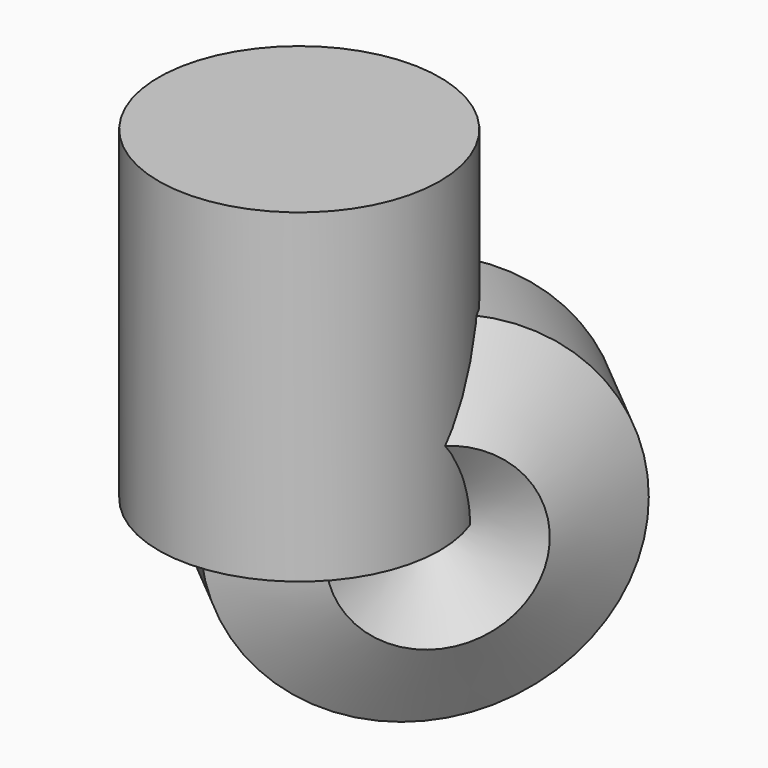
from build123d import *

# Parameters (mm, degrees)
F0_R     = 54.9531653684
F1_DEPTH = 127
F7_DEPTH = 25.4


# Not quite as in the source:
# - a feature of the source that left no trace in its solid (it failed there, or was rolled back) is left out
# - the program builds the solid bodies; features that only make, move or delete a surface that nothing else refers to are left out


with BuildPart() as f1:
    # F0 (on Top) → F1 (new body)
    with BuildSketch(Plane.XY):
        Circle(F0_R)
    extrude(amount=F1_DEPTH)


with BuildPart() as f3:
    # F2 (on Top) → F3 (revolve)
    with BuildSketch(Plane.XY):
        Polygon((30.9442904428, -25.8326890354), (37.8439101741, 13.8821971078), (6.8996197313, 39.7148861432), (-30.9442904428, 25.8326890354), (-37.8439101741, -13.8821971078), (-6.8996197313, -39.7148861432), align=None)
    revolve(axis=Axis((22.3717649527, 26.7985416255, 0), (0.7676624397, -0.640854413, 0)))


with BuildPart() as f7:
    # F6 (on Top) → F7 (new body)
    with BuildSketch(Plane.XY):
        with BuildLine():
            add(Edge.make_bspline(
                [(-22.4183332175, 16.1747615784), (-11.8871169461, 25.9707679053), (-5.6486125726, 51.1465707181), (42.7874188306, 27.4433614183), (39.8462276715, -30.123574606), (-2.9479560075, -20.4408335204), (-31.1948387365, -43.0855866328), (-18.3031677908, -3.1092882088), (-65.8787672835, -7.2071620203), (-32.9625958172, 6.3666197193), (-22.4183332175, 16.1747615784)],
                knots=[0, 0, 0, 0, 0.1298859642, 0.2693514147, 0.414375979, 0.5513899534, 0.6555656862, 0.7633147629, 0.8699531299, 1, 1, 1, 1], degree=3))
        make_face()
    extrude(amount=F7_DEPTH)


solid = Compound([f1.part, f3.part, f7.part])
